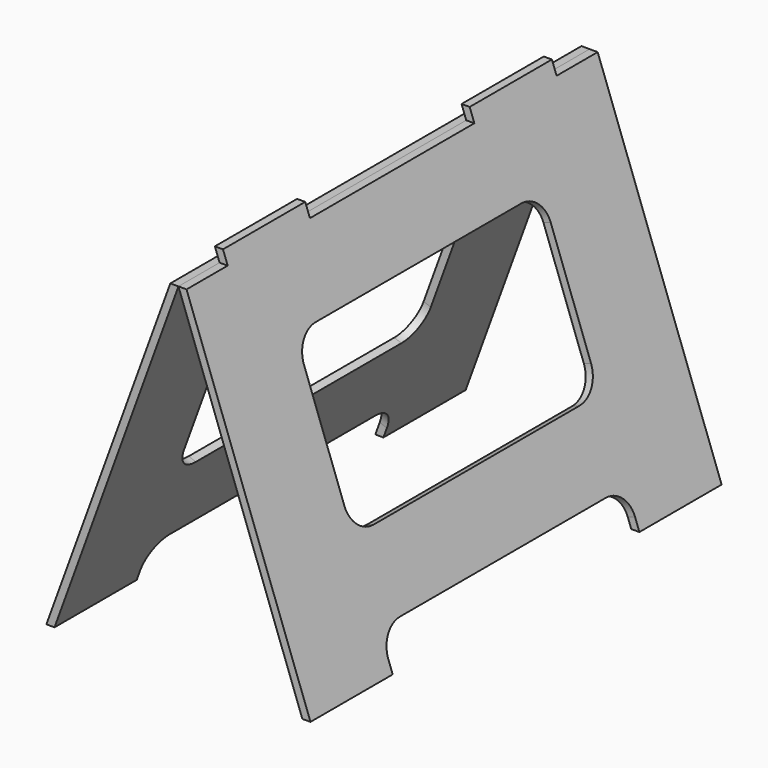
from build123d import *

# Parameters (mm, degrees)
F1_DEPTH  = 508
F2_DEPTH  = 508
F3_W      = 203.2
F3_H      = 25.4
F3_W_2    = 101.6
F4_DEPTH  = 25.4
F6_DEPTH  = 490.591016945
F8_DEPTH  = 490.591016945
F10_DEPTH = 490.591016945


with BuildPart() as f1:
    # F0 (on Front) → F1 (new body, symmetric)
    with BuildSketch(Plane.XZ):
        Polygon((6.8042870808, 25.4), (-9.2448439504, 25.4), (0, 0), (244.9883646846, -673.1), (261.0374957157, -673.1), align=None)
    extrude(amount=F1_DEPTH, both=True)

    # F3 (on Right) → F4 (cut, symmetric)
    with BuildSketch(Plane.YZ):
        with Locations((-101.6, 12.7)):
            Rectangle(F3_W, F3_H)
        with Locations((101.6, 12.7)):
            Rectangle(F3_W, F3_H)
        with Locations((-457.2, 12.7)):
            Rectangle(F3_W_2, F3_H)
        with Locations((457.2, 12.7)):
            Rectangle(F3_W_2, F3_H)
    extrude(amount=F4_DEPTH, both=True, mode=Mode.SUBTRACT)

    # F5 (on face) → F6 (cut, through all)
    with BuildSketch(Plane(origin=(14.1717393372, 0, 5.1580912865), x_dir=(0, 1, 0), z_dir=(0.9396926208, 0, 0.3420201433))):
        with BuildLine():
            Line((-304.8, -696.3871847491), (-304.8, -721.7871847491))
            Line((-304.8, -721.7871847491), (304.8, -721.7871847491))
            Line((304.8, -721.7871847491), (304.8, -696.3871847491))
            ThreePointArc((304.8, -696.3871847491), (289.9210244843, -660.4661602648), (254, -645.5871847491))
            Line((254, -645.5871847491), (-254, -645.5871847491))
            ThreePointArc((-254, -645.5871847491), (-289.9210244843, -660.4661602648), (-304.8, -696.3871847491))
        make_face()
    extrude(amount=-F6_DEPTH, mode=Mode.SUBTRACT)

    # F7 (on face) → F8 (cut, through all)
    with BuildSketch(Plane(origin=(14.1717393372, 0, 5.1580912865), x_dir=(0, 1, 0), z_dir=(0.9396926208, 0, 0.3420201433))):
        with BuildLine():
            Line((254, -157.8891260955), (-254, -157.8891260955))
            ThreePointArc((-254, -157.8891260955), (-289.9210244843, -172.7681016113), (-304.8, -208.6891260955))
            Line((-304.8, -208.6891260955), (-304.8, -442.3871847491))
            ThreePointArc((-304.8, -442.3871847491), (-289.9210244843, -478.3082092333), (-254, -493.1871847491))
            Line((-254, -493.1871847491), (254, -493.1871847491))
            ThreePointArc((254, -493.1871847491), (289.9210244843, -478.3082092333), (304.8, -442.3871847491))
            Line((304.8, -442.3871847491), (304.8, -208.6891260955))
            ThreePointArc((304.8, -208.6891260955), (289.9210244843, -172.7681016113), (254, -157.8891260955))
        make_face()
    extrude(amount=-F8_DEPTH, mode=Mode.SUBTRACT)


with BuildPart() as f2:
    # F0 (on Front) → F2 (new body, symmetric)
    with BuildSketch(Plane.XZ):
        Polygon((-244.9883646846, -673.1), (0, 0), (-16.0491310312, 0), (-261.0374957157, -673.1), align=None)
    extrude(amount=F2_DEPTH, both=True)

    # F9 (on face) → F10 (cut, through all)
    with BuildSketch(Plane(origin=(-14.1717393372, 0, 5.1580912865), x_dir=(0, -1, 0), z_dir=(-0.9396926208, 0, 0.3420201433))):
        with BuildLine():
            Line((254, -157.8891260955), (-254, -157.8891260955))
            ThreePointArc((-254, -157.8891260955), (-289.9210244843, -172.7681016113), (-304.8, -208.6891260955))
            Line((-304.8, -208.6891260955), (-304.8, -442.3871847491))
            ThreePointArc((-304.8, -442.3871847491), (-289.9210244843, -478.3082092333), (-254, -493.1871847491))
            Line((-254, -493.1871847491), (254, -493.1871847491))
            ThreePointArc((254, -493.1871847491), (289.9210244843, -478.3082092333), (304.8, -442.3871847491))
            Line((304.8, -442.3871847491), (304.8, -208.6891260955))
            ThreePointArc((304.8, -208.6891260955), (289.9210244843, -172.7681016113), (254, -157.8891260955))
        make_face()
        with BuildLine():
            Line((-304.8, -696.3871847491), (-304.8, -721.7871847491))
            Line((-304.8, -721.7871847491), (304.8, -721.7871847491))
            Line((304.8, -721.7871847491), (304.8, -696.3871847491))
            ThreePointArc((304.8, -696.3871847491), (289.9210244843, -660.4661602648), (254, -645.5871847491))
            Line((254, -645.5871847491), (-254, -645.5871847491))
            ThreePointArc((-254, -645.5871847491), (-289.9210244843, -660.4661602648), (-304.8, -696.3871847491))
        make_face()
    extrude(amount=-F10_DEPTH, mode=Mode.SUBTRACT)


solid = Compound([f1.part, f2.part])
